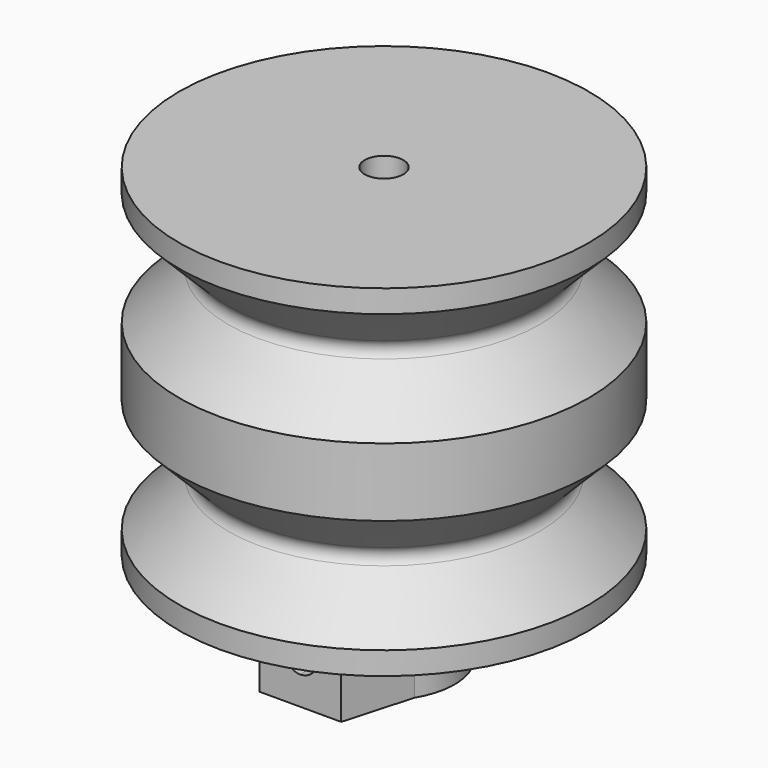
from build123d import *

# Parameters (mm, degrees)
F1_DEPTH     = 8
F3_W         = 6.7527772065
F3_H         = 8
F4_DEPTH     = 4
F8_DEPTH     = 7
F9_T4_DEPTH  = 8
F9_T9_DEPTH  = 20.6550440955
F9_T15_DEPTH = 20.6550440955
F9_T21_DEPTH = 8
F9_T26_DEPTH = 20.6550440955
F9_T32_DEPTH = 20.6550440955
F12_DEPTH    = 8
F13_SIZE     = 3.5
F16_R        = 1
F17_DEPTH    = 5
F20_R        = 1
F21_DEPTH    = 5


# Not quite as in the source:
# - a fillet or chamfer that OpenCascade refuses, or shapes differently, is made with other operations: its cross-section is extruded or revolved along the edge and cut away or added


with BuildPart() as f1:
    # F0 (on Top) → F1 (new body)
    with BuildSketch(Plane.XY):
        with BuildLine():
            Line((-3.3763886032, -5.2), (3.3763886032, -5.2))
            ThreePointArc((3.3763886032, -5.2), (0, 6.2), (-3.3763886032, -5.2))
        make_face()
        with BuildLine():
            ThreePointArc((-1.8439088915, -1.2), (0, 2.2), (1.8439088915, -1.2))
            Line((1.8439088915, -1.2), (-1.8439088915, -1.2))
        make_face(mode=Mode.SUBTRACT)
    extrude(amount=F1_DEPTH)

    # F3 (on offset) → F4 (join)
    with BuildSketch(Plane.XZ.offset(5.2)):
        with Locations((0, 4)):
            Rectangle(F3_W, F3_H)
    extrude(amount=F4_DEPTH)

    # F6 (on Right) → F7 (revolve)
    with BuildSketch(Plane.YZ):
        with BuildLine():
            Line((18, 36), (18, 38))
            Line((18, 38), (1.7, 38))
            Line((1.7, 38), (1.7, 34))
            Line((1.7, 34), (0, 31.9740188926))
            Line((0, 31.9740188926), (0, 8))
            Line((0, 8), (18, 8))
            Line((18, 8), (18, 10))
            Line((18, 10), (13.7071067812, 14.2928932188))
            ThreePointArc((13.7071067812, 14.2928932188), (13.4142135624, 15), (13.7071067812, 15.7071067812))
            Line((13.7071067812, 15.7071067812), (18, 20))
            Line((18, 20), (18, 26))
            Line((18, 26), (13.7071067812, 30.2928932188))
            ThreePointArc((13.7071067812, 30.2928932188), (13.4142135624, 31), (13.7071067812, 31.7071067812))
            Line((13.7071067812, 31.7071067812), (18, 36))
        make_face()
    revolve(axis=Axis((0, 0, 19.9870094463), (0, 0, 1)))

    # F5 (on Top) → F8 (cut)
    with BuildSketch(Plane.XY):
        Polygon((3, -5.5), (3, -3), (0, -3), (-3, -3), (-3, -5.5), align=None)
    extrude(amount=F8_DEPTH, mode=Mode.SUBTRACT)

    # F9: chamfer of 7 on 2 edges, made by hand


with BuildPart() as f9_tool2:
    # F9_s3 → F9_t4 (new body)
    with BuildSketch(Plane.XY):
        with BuildLine():
            Line((-3.3002459804, -10.261444939), (-5.3591596162, -2.9755066267))
            Line((-5.3591596162, -2.9755066267), (-5.2398656841, -2.9022334545))
            ThreePointArc((-5.2398656841, -2.9022334545), (-4.424549602, -4.1408888924), (-3.3001475703, -5.0825806452))
            Line((-3.3001475703, -5.0825806452), (-3.2363886032, -5.2))
            ThreePointArc((-3.2363886032, -5.2), (-3.2363886032, -7.7307224695), (-3.1602459804, -10.261444939))
            Line((-3.1602459804, -10.261444939), (-3.3002459804, -10.261444939))
        make_face()
    extrude(amount=F9_T4_DEPTH)

    split(bisect_by=Plane.XZ.offset(9.2), keep=Keep.BOTTOM)


with BuildPart() as f1_1:
    add(f1.part)

    # F9_t1: union F9_tool2
    add(f9_tool2.part)


with BuildPart() as f9_tool7:
    # F9_s8 → F9_t9 (new body)
    with BuildSketch(Plane.XY):
        with BuildLine():
            Line((-3.3002459804, -10.261444939), (-5.3591596162, -2.9755066267))
            Line((-5.3591596162, -2.9755066267), (-5.2398656841, -2.9022334545))
            ThreePointArc((-5.2398656841, -2.9022334545), (-4.424549602, -4.1408888924), (-3.3001475703, -5.0825806452))
            Line((-3.3001475703, -5.0825806452), (-3.2363886032, -5.2))
            ThreePointArc((-3.2363886032, -5.2), (-3.2363886032, -7.7307224695), (-3.1602459804, -10.261444939))
            Line((-3.1602459804, -10.261444939), (-3.3002459804, -10.261444939))
        make_face()
    extrude(amount=F9_T9_DEPTH)

    split(bisect_by=Plane.XY.offset(8), keep=Keep.TOP)

    split(bisect_by=Plane.XZ.offset(9.2), keep=Keep.TOP)


with BuildPart() as f1_2:
    add(f1_1.part)

    # F9_t6: union F9_tool7
    add(f9_tool7.part)


with BuildPart() as f9_tool13:
    # F9_s14 → F9_t15 (new body)
    with BuildSketch(Plane.XY):
        with BuildLine():
            Line((-3.3002459804, -10.261444939), (-5.3591596162, -2.9755066267))
            Line((-5.3591596162, -2.9755066267), (-5.2398656841, -2.9022334545))
            ThreePointArc((-5.2398656841, -2.9022334545), (-4.424549602, -4.1408888924), (-3.3001475703, -5.0825806452))
            Line((-3.3001475703, -5.0825806452), (-3.2363886032, -5.2))
            ThreePointArc((-3.2363886032, -5.2), (-3.2363886032, -7.7307224695), (-3.1602459804, -10.261444939))
            Line((-3.1602459804, -10.261444939), (-3.3002459804, -10.261444939))
        make_face()
    extrude(amount=F9_T15_DEPTH)

    split(bisect_by=Plane.XY.offset(8), keep=Keep.TOP)

    split(bisect_by=Plane.XZ.offset(9.2), keep=Keep.BOTTOM)


with BuildPart() as f1_3:
    add(f1_2.part)

    # F9_t12: union F9_tool13
    add(f9_tool13.part)


with BuildPart() as f9_tool19:
    # F9_s20 → F9_t21 (new body)
    with BuildSketch(Plane.XY):
        with BuildLine():
            Line((3.3002459804, -10.261444939), (5.3591596162, -2.9755066267))
            Line((5.3591596162, -2.9755066267), (5.2398656841, -2.9022334545))
            ThreePointArc((5.2398656841, -2.9022334545), (4.424549602, -4.1408888924), (3.3001475703, -5.0825806452))
            Line((3.3001475703, -5.0825806452), (3.2363886032, -5.2))
            ThreePointArc((3.2363886032, -5.2), (3.2363886032, -7.7307224695), (3.1602459804, -10.261444939))
            Line((3.1602459804, -10.261444939), (3.3002459804, -10.261444939))
        make_face()
    extrude(amount=F9_T21_DEPTH)

    split(bisect_by=Plane.XZ.offset(9.2), keep=Keep.BOTTOM)


with BuildPart() as f1_4:
    add(f1_3.part)

    # F9_t18: union F9_tool19
    add(f9_tool19.part)


with BuildPart() as f9_tool24:
    # F9_s25 → F9_t26 (new body)
    with BuildSketch(Plane.XY):
        with BuildLine():
            Line((3.3002459804, -10.261444939), (5.3591596162, -2.9755066267))
            Line((5.3591596162, -2.9755066267), (5.2398656841, -2.9022334545))
            ThreePointArc((5.2398656841, -2.9022334545), (4.424549602, -4.1408888924), (3.3001475703, -5.0825806452))
            Line((3.3001475703, -5.0825806452), (3.2363886032, -5.2))
            ThreePointArc((3.2363886032, -5.2), (3.2363886032, -7.7307224695), (3.1602459804, -10.261444939))
            Line((3.1602459804, -10.261444939), (3.3002459804, -10.261444939))
        make_face()
    extrude(amount=F9_T26_DEPTH)

    split(bisect_by=Plane.XY.offset(8), keep=Keep.TOP)

    split(bisect_by=Plane.XZ.offset(9.2), keep=Keep.TOP)


with BuildPart() as f1_5:
    add(f1_4.part)

    # F9_t23: union F9_tool24
    add(f9_tool24.part)


with BuildPart() as f9_tool30:
    # F9_s31 → F9_t32 (new body)
    with BuildSketch(Plane.XY):
        with BuildLine():
            Line((3.3002459804, -10.261444939), (5.3591596162, -2.9755066267))
            Line((5.3591596162, -2.9755066267), (5.2398656841, -2.9022334545))
            ThreePointArc((5.2398656841, -2.9022334545), (4.424549602, -4.1408888924), (3.3001475703, -5.0825806452))
            Line((3.3001475703, -5.0825806452), (3.2363886032, -5.2))
            ThreePointArc((3.2363886032, -5.2), (3.2363886032, -7.7307224695), (3.1602459804, -10.261444939))
            Line((3.1602459804, -10.261444939), (3.3002459804, -10.261444939))
        make_face()
    extrude(amount=F9_T32_DEPTH)

    split(bisect_by=Plane.XY.offset(8), keep=Keep.TOP)

    split(bisect_by=Plane.XZ.offset(9.2), keep=Keep.BOTTOM)


with BuildPart() as f1_6:
    add(f1_5.part)

    # F9_t29: union F9_tool30
    add(f9_tool30.part)

    # F11 (on offset) → F12 (cut, through all)
    with BuildSketch(Plane.XZ.offset(9.2)):
        with BuildLine():
            ThreePointArc((0, 2.5), (1.0606601718, 2.9393398282), (1.5, 4))
            ThreePointArc((1.5, 4), (-1.0606601718, 5.0606601718), (0, 2.5))
        make_face()
    extrude(amount=-F12_DEPTH, mode=Mode.SUBTRACT)

    # F13
    f13_edges = [f1_6.edges().sort_by_distance(p)[0] for p in [
        (0, 6.2, 8),
    ]]
    chamfer(f13_edges, length=F13_SIZE)

    # F16 (on face) → F17 (cut)
    with BuildSketch(Plane(origin=(0, -1, 1), x_dir=(1, 0, 0), z_dir=(0, -0.7071067812, 0.7071067812))):
        with Locations((0, 23.2666600496)):
            Circle(F16_R)
    extrude(amount=F17_DEPTH, mode=Mode.SUBTRACT)

    # F20 (on face) → F21 (cut)
    with BuildSketch(Plane(origin=(0, -9, 9), x_dir=(1, 0, 0), z_dir=(0, -0.7071067812, 0.7071067812))):
        with Locations((0, 33.659003675)):
            Circle(F20_R)
    extrude(amount=F21_DEPTH, mode=Mode.SUBTRACT)


solid = f1_6.part
